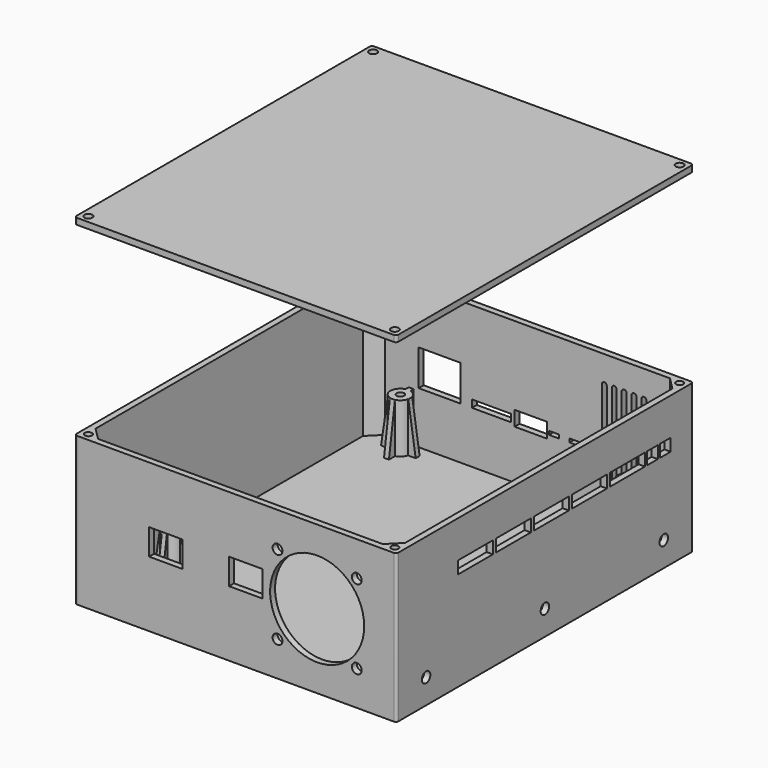
from build123d import *

# Parameters (mm, degrees)
F0_R        = 1.5
F1_DEPTH    = 60
F2_T        = -2.5
F3_DEPTH    = 22.5
F4_W        = 17
F4_H        = 14.5
F4_W_2      = 15.8
F4_H_2      = 3
F4_W_3      = 13
F4_H_3      = 6
F4_W_4      = 4
F4_H_4      = 1.45
F5_DEPTH    = 2.5
F6_R        = 19
F6_R_2      = 2
F6_W        = 13.5
F6_H        = 10.5
F7_DEPTH    = 2.5
F8_R        = 2.15
F8_W        = 17.7
F8_H        = 5
F8_W_2      = 5.5
F9_DEPTH    = 2.5
F12_DEPTH   = 2.5
F13_SIZE2   = 19.99999
F13_SIZE    = 2.99999
F14_SIZE2   = 2.99999
F14_SIZE    = 19.99999
F14_2_SIZE2 = 2.99999
F14_2_SIZE  = 19.99999
F14_3_SIZE2 = 2.99999
F14_3_SIZE  = 19.99999
F14_4_SIZE2 = 2.99999
F14_4_SIZE  = 19.99999
F14_5_SIZE2 = 2.99999
F14_5_SIZE  = 19.99999
F14_6_SIZE2 = 2.99999
F14_6_SIZE  = 19.99999
F14_7_SIZE2 = 2.99999
F14_7_SIZE  = 19.99999
F15_SIZE2   = 19.99999
F15_SIZE    = 2.99999
F15_2_SIZE2 = 19.99999
F15_2_SIZE  = 2.99999
F16_DEPTH   = 60
F17_R       = 1.45
F18_DEPTH   = 15
F19_W       = 130
F19_H       = 150
F20_DEPTH   = 2.5
F22_R       = 1.6
F23_DEPTH   = 2.5
F24_R       = 1
F24_2_R     = 1


# Not quite as in the source:
# - a fillet or chamfer is up to 0.001 mm smaller than in the source, because OpenCascade refuses the exact size


with BuildPart() as f1:
    # F0 (on Top) → F1 (new body)
    with BuildSketch(Plane.XY):
        Polygon((-55, -75), (55, -75), (65, -65), (65, 65), (55, 75), (-55, 75), (-65, 65), (-65, -65), align=None)
        with BuildLine():
            ThreePointArc((-46, -44.1270166538), (-44.1715728753, -45.1715728753), (-43.1270166538, -47))
            Line((-43.1270166538, -47), (-40, -47))
            Line((-40, -47), (-40, -49))
            Line((-40, -49), (-43.1270166538, -49))
            ThreePointArc((-43.1270166538, -49), (-44.1715728753, -50.8284271247), (-46, -51.8729833462))
            Line((-46, -51.8729833462), (-46, -55))
            Line((-46, -55), (-48, -55))
            Line((-48, -55), (-48, -51.8729833462))
            ThreePointArc((-48, -51.8729833462), (-49.8284271247, -50.8284271247), (-50.8729833462, -49))
            Line((-50.8729833462, -49), (-54, -49))
            Line((-54, -49), (-54, -47))
            Line((-54, -47), (-50.8729833462, -47))
            ThreePointArc((-50.8729833462, -47), (-49.8284271247, -45.1715728753), (-48, -44.1270166538))
            Line((-48, -44.1270166538), (-48, -41))
            Line((-48, -41), (-46, -41))
            Line((-46, -41), (-46, -44.1270166538))
        make_face(mode=Mode.SUBTRACT)
        with BuildLine():
            ThreePointArc((46, -44.1270166538), (47.8284271247, -45.1715728753), (48.8729833462, -47))
            Line((48.8729833462, -47), (52, -47))
            Line((52, -47), (52, -49))
            Line((52, -49), (48.8729833462, -49))
            ThreePointArc((48.8729833462, -49), (47.8284271247, -50.8284271247), (46, -51.8729833462))
            Line((46, -51.8729833462), (46, -55))
            Line((46, -55), (44, -55))
            Line((44, -55), (44, -51.8729833462))
            ThreePointArc((44, -51.8729833462), (42.1715728753, -50.8284271247), (41.1270166538, -49))
            Line((41.1270166538, -49), (38, -49))
            Line((38, -49), (38, -47))
            Line((38, -47), (41.1270166538, -47))
            ThreePointArc((41.1270166538, -47), (42.1715728753, -45.1715728753), (44, -44.1270166538))
            Line((44, -44.1270166538), (44, -41))
            Line((44, -41), (46, -41))
            Line((46, -41), (46, -44.1270166538))
        make_face(mode=Mode.SUBTRACT)
        with BuildLine():
            ThreePointArc((-46, 70.8729833462), (-44.1715728753, 69.8284271247), (-43.1270166538, 68))
            Line((-43.1270166538, 68), (-40, 68))
            Line((-40, 68), (-40, 66))
            Line((-40, 66), (-43.1270166538, 66))
            ThreePointArc((-43.1270166538, 66), (-44.1715728753, 64.1715728753), (-46, 63.1270166538))
            Line((-46, 63.1270166538), (-46, 60))
            Line((-46, 60), (-48, 60))
            Line((-48, 60), (-48, 63.1270166538))
            ThreePointArc((-48, 63.1270166538), (-49.8284271247, 64.1715728753), (-50.8729833462, 66))
            Line((-50.8729833462, 66), (-54, 66))
            Line((-54, 66), (-54, 68))
            Line((-54, 68), (-50.8729833462, 68))
            ThreePointArc((-50.8729833462, 68), (-49.8284271247, 69.8284271247), (-48, 70.8729833462))
            Line((-48, 70.8729833462), (-48, 74))
            Line((-48, 74), (-46, 74))
            Line((-46, 74), (-46, 70.8729833462))
        make_face(mode=Mode.SUBTRACT)
        with BuildLine():
            ThreePointArc((46, 70.8729833462), (47.8284271247, 69.8284271247), (48.8729833462, 68))
            Line((48.8729833462, 68), (52, 68))
            Line((52, 68), (52, 66))
            Line((52, 66), (48.8729833462, 66))
            ThreePointArc((48.8729833462, 66), (47.8284271247, 64.1715728753), (46, 63.1270166538))
            Line((46, 63.1270166538), (46, 60))
            Line((46, 60), (44, 60))
            Line((44, 60), (44, 63.1270166538))
            ThreePointArc((44, 63.1270166538), (42.1715728753, 64.1715728753), (41.1270166538, 66))
            Line((41.1270166538, 66), (38, 66))
            Line((38, 66), (38, 68))
            Line((38, 68), (41.1270166538, 68))
            ThreePointArc((41.1270166538, 68), (42.1715728753, 69.8284271247), (44, 70.8729833462))
            Line((44, 70.8729833462), (44, 74))
            Line((44, 74), (46, 74))
            Line((46, 74), (46, 70.8729833462))
        make_face(mode=Mode.SUBTRACT)
        with BuildLine():
            ThreePointArc((48.8729833462, 66), (48.9681187851, 66.4959828301), (49, 67))
            ThreePointArc((49, 67), (48.9681187851, 67.5040171699), (48.8729833462, 68))
            ThreePointArc((48.8729833462, 68), (47.8284271247, 69.8284271247), (46, 70.8729833462))
            ThreePointArc((46, 70.8729833462), (45, 71), (44, 70.8729833462))
            ThreePointArc((44, 70.8729833462), (42.1715728753, 69.8284271247), (41.1270166538, 68))
            ThreePointArc((41.1270166538, 68), (41, 67), (41.1270166538, 66))
            ThreePointArc((41.1270166538, 66), (42.1715728753, 64.1715728753), (44, 63.1270166538))
            ThreePointArc((44, 63.1270166538), (45, 63), (46, 63.1270166538))
            ThreePointArc((46, 63.1270166538), (47.8284271247, 64.1715728753), (48.8729833462, 66))
        make_face()
        with Locations((45, 67)):
            Circle(F0_R, mode=Mode.SUBTRACT)
        with BuildLine():
            ThreePointArc((-43.1270166538, -49), (-43.0318812149, -48.5040171699), (-43, -48))
            ThreePointArc((-43, -48), (-43.0318812149, -47.4959828301), (-43.1270166538, -47))
            ThreePointArc((-43.1270166538, -47), (-44.1715728753, -45.1715728753), (-46, -44.1270166538))
            ThreePointArc((-46, -44.1270166538), (-47, -44), (-48, -44.1270166538))
            ThreePointArc((-48, -44.1270166538), (-49.8284271247, -45.1715728753), (-50.8729833462, -47))
            ThreePointArc((-50.8729833462, -47), (-51, -48), (-50.8729833462, -49))
            ThreePointArc((-50.8729833462, -49), (-49.8284271247, -50.8284271247), (-48, -51.8729833462))
            ThreePointArc((-48, -51.8729833462), (-47, -52), (-46, -51.8729833462))
            ThreePointArc((-46, -51.8729833462), (-44.1715728753, -50.8284271247), (-43.1270166538, -49))
        make_face()
        with Locations((-47, -48)):
            Circle(F0_R, mode=Mode.SUBTRACT)
        with BuildLine():
            ThreePointArc((-43.1270166538, 66), (-43.0318812149, 66.4959828301), (-43, 67))
            ThreePointArc((-43, 67), (-43.0318812149, 67.5040171699), (-43.1270166538, 68))
            ThreePointArc((-43.1270166538, 68), (-44.1715728753, 69.8284271247), (-46, 70.8729833462))
            ThreePointArc((-46, 70.8729833462), (-47, 71), (-48, 70.8729833462))
            ThreePointArc((-48, 70.8729833462), (-49.8284271247, 69.8284271247), (-50.8729833462, 68))
            ThreePointArc((-50.8729833462, 68), (-51, 67), (-50.8729833462, 66))
            ThreePointArc((-50.8729833462, 66), (-49.8284271247, 64.1715728753), (-48, 63.1270166538))
            ThreePointArc((-48, 63.1270166538), (-47, 63), (-46, 63.1270166538))
            ThreePointArc((-46, 63.1270166538), (-44.1715728753, 64.1715728753), (-43.1270166538, 66))
        make_face()
        with Locations((-47, 67)):
            Circle(F0_R, mode=Mode.SUBTRACT)
        with BuildLine():
            ThreePointArc((48.8729833462, -49), (48.9681187851, -48.5040171699), (49, -48))
            ThreePointArc((49, -48), (48.9681187851, -47.4959828301), (48.8729833462, -47))
            ThreePointArc((48.8729833462, -47), (47.8284271247, -45.1715728753), (46, -44.1270166538))
            ThreePointArc((46, -44.1270166538), (45, -44), (44, -44.1270166538))
            ThreePointArc((44, -44.1270166538), (42.1715728753, -45.1715728753), (41.1270166538, -47))
            ThreePointArc((41.1270166538, -47), (41, -48), (41.1270166538, -49))
            ThreePointArc((41.1270166538, -49), (42.1715728753, -50.8284271247), (44, -51.8729833462))
            ThreePointArc((44, -51.8729833462), (45, -52), (46, -51.8729833462))
            ThreePointArc((46, -51.8729833462), (47.8284271247, -50.8284271247), (48.8729833462, -49))
        make_face()
        with Locations((45, -48)):
            Circle(F0_R, mode=Mode.SUBTRACT)
        Polygon((55, -75), (65, -75), (65, -65), align=None)
        Polygon((-65, -75), (-55, -75), (-65, -65), align=None)
        Polygon((55, 75), (65, 65), (65, 75), align=None)
        Polygon((-65, 75), (-65, 65), (-55, 75), align=None)
        with Locations((45, 67)):
            Circle(F0_R)
        with Locations((-47, 67)):
            Circle(F0_R)
        with Locations((-47, -48)):
            Circle(F0_R)
        with Locations((45, -48)):
            Circle(F0_R)
        with BuildLine():
            Line((-46, 60), (-46, 63.1270166538))
            ThreePointArc((-46, 63.1270166538), (-47, 63), (-48, 63.1270166538))
            Line((-48, 63.1270166538), (-48, 60))
            Line((-48, 60), (-46, 60))
        make_face()
        with BuildLine():
            ThreePointArc((-50.8729833462, -49), (-51, -48), (-50.8729833462, -47))
            Line((-50.8729833462, -47), (-54, -47))
            Line((-54, -47), (-54, -49))
            Line((-54, -49), (-50.8729833462, -49))
        make_face()
        with BuildLine():
            Line((-46, -55), (-46, -51.8729833462))
            ThreePointArc((-46, -51.8729833462), (-47, -52), (-48, -51.8729833462))
            Line((-48, -51.8729833462), (-48, -55))
            Line((-48, -55), (-46, -55))
        make_face()
        with BuildLine():
            ThreePointArc((-50.8729833462, 66), (-51, 67), (-50.8729833462, 68))
            Line((-50.8729833462, 68), (-54, 68))
            Line((-54, 68), (-54, 66))
            Line((-54, 66), (-50.8729833462, 66))
        make_face()
        with BuildLine():
            Line((46, -55), (46, -51.8729833462))
            ThreePointArc((46, -51.8729833462), (45, -52), (44, -51.8729833462))
            Line((44, -51.8729833462), (44, -55))
            Line((44, -55), (46, -55))
        make_face()
        with BuildLine():
            ThreePointArc((48.8729833462, 68), (48.9681187851, 67.5040171699), (49, 67))
            ThreePointArc((49, 67), (48.9681187851, 66.4959828301), (48.8729833462, 66))
            Line((48.8729833462, 66), (52, 66))
            Line((52, 66), (52, 68))
            Line((52, 68), (48.8729833462, 68))
        make_face()
        with BuildLine():
            Line((46, 60), (46, 63.1270166538))
            ThreePointArc((46, 63.1270166538), (45, 63), (44, 63.1270166538))
            Line((44, 63.1270166538), (44, 60))
            Line((44, 60), (46, 60))
        make_face()
        with BuildLine():
            ThreePointArc((-43.1270166538, -47), (-43.0318812149, -47.4959828301), (-43, -48))
            ThreePointArc((-43, -48), (-43.0318812149, -48.5040171699), (-43.1270166538, -49))
            Line((-43.1270166538, -49), (-40, -49))
            Line((-40, -49), (-40, -47))
            Line((-40, -47), (-43.1270166538, -47))
        make_face()
        with BuildLine():
            ThreePointArc((44, -44.1270166538), (45, -44), (46, -44.1270166538))
            Line((46, -44.1270166538), (46, -41))
            Line((46, -41), (44, -41))
            Line((44, -41), (44, -44.1270166538))
        make_face()
        with BuildLine():
            ThreePointArc((41.1270166538, -49), (41, -48), (41.1270166538, -47))
            Line((41.1270166538, -47), (38, -47))
            Line((38, -47), (38, -49))
            Line((38, -49), (41.1270166538, -49))
        make_face()
        with BuildLine():
            ThreePointArc((-48, -44.1270166538), (-47, -44), (-46, -44.1270166538))
            Line((-46, -44.1270166538), (-46, -41))
            Line((-46, -41), (-48, -41))
            Line((-48, -41), (-48, -44.1270166538))
        make_face()
        with BuildLine():
            ThreePointArc((-43.1270166538, 68), (-43.0318812149, 67.5040171699), (-43, 67))
            ThreePointArc((-43, 67), (-43.0318812149, 66.4959828301), (-43.1270166538, 66))
            Line((-43.1270166538, 66), (-40, 66))
            Line((-40, 66), (-40, 68))
            Line((-40, 68), (-43.1270166538, 68))
        make_face()
        with BuildLine():
            ThreePointArc((44, 70.8729833462), (45, 71), (46, 70.8729833462))
            Line((46, 70.8729833462), (46, 74))
            Line((46, 74), (44, 74))
            Line((44, 74), (44, 70.8729833462))
        make_face()
        with BuildLine():
            ThreePointArc((48.8729833462, -47), (48.9681187851, -47.4959828301), (49, -48))
            ThreePointArc((49, -48), (48.9681187851, -48.5040171699), (48.8729833462, -49))
            Line((48.8729833462, -49), (52, -49))
            Line((52, -49), (52, -47))
            Line((52, -47), (48.8729833462, -47))
        make_face()
        with BuildLine():
            ThreePointArc((41.1270166538, 66), (41, 67), (41.1270166538, 68))
            Line((41.1270166538, 68), (38, 68))
            Line((38, 68), (38, 66))
            Line((38, 66), (41.1270166538, 66))
        make_face()
        with BuildLine():
            ThreePointArc((-48, 70.8729833462), (-47, 71), (-46, 70.8729833462))
            Line((-46, 70.8729833462), (-46, 74))
            Line((-46, 74), (-48, 74))
            Line((-48, 74), (-48, 70.8729833462))
        make_face()
    extrude(amount=F1_DEPTH)

    # F2
    f2_openings = [f1.faces().sort_by_distance(p)[0] for p in [
        (0, 0, 60),
    ]]
    offset(amount=F2_T, openings=f2_openings)

    # F0 (on Top) → F3 (join)
    with BuildSketch(Plane.XY):
        with BuildLine():
            ThreePointArc((-43.1270166538, 66), (-43.0318812149, 66.4959828301), (-43, 67))
            ThreePointArc((-43, 67), (-43.0318812149, 67.5040171699), (-43.1270166538, 68))
            ThreePointArc((-43.1270166538, 68), (-44.1715728753, 69.8284271247), (-46, 70.8729833462))
            ThreePointArc((-46, 70.8729833462), (-47, 71), (-48, 70.8729833462))
            ThreePointArc((-48, 70.8729833462), (-49.8284271247, 69.8284271247), (-50.8729833462, 68))
            ThreePointArc((-50.8729833462, 68), (-51, 67), (-50.8729833462, 66))
            ThreePointArc((-50.8729833462, 66), (-49.8284271247, 64.1715728753), (-48, 63.1270166538))
            ThreePointArc((-48, 63.1270166538), (-47, 63), (-46, 63.1270166538))
            ThreePointArc((-46, 63.1270166538), (-44.1715728753, 64.1715728753), (-43.1270166538, 66))
        make_face()
        with Locations((-47, 67)):
            Circle(F0_R, mode=Mode.SUBTRACT)
        with BuildLine():
            ThreePointArc((-43.1270166538, -49), (-43.0318812149, -48.5040171699), (-43, -48))
            ThreePointArc((-43, -48), (-43.0318812149, -47.4959828301), (-43.1270166538, -47))
            ThreePointArc((-43.1270166538, -47), (-44.1715728753, -45.1715728753), (-46, -44.1270166538))
            ThreePointArc((-46, -44.1270166538), (-47, -44), (-48, -44.1270166538))
            ThreePointArc((-48, -44.1270166538), (-49.8284271247, -45.1715728753), (-50.8729833462, -47))
            ThreePointArc((-50.8729833462, -47), (-51, -48), (-50.8729833462, -49))
            ThreePointArc((-50.8729833462, -49), (-49.8284271247, -50.8284271247), (-48, -51.8729833462))
            ThreePointArc((-48, -51.8729833462), (-47, -52), (-46, -51.8729833462))
            ThreePointArc((-46, -51.8729833462), (-44.1715728753, -50.8284271247), (-43.1270166538, -49))
        make_face()
        with Locations((-47, -48)):
            Circle(F0_R, mode=Mode.SUBTRACT)
        with BuildLine():
            ThreePointArc((48.8729833462, -49), (48.9681187851, -48.5040171699), (49, -48))
            ThreePointArc((49, -48), (48.9681187851, -47.4959828301), (48.8729833462, -47))
            ThreePointArc((48.8729833462, -47), (47.8284271247, -45.1715728753), (46, -44.1270166538))
            ThreePointArc((46, -44.1270166538), (45, -44), (44, -44.1270166538))
            ThreePointArc((44, -44.1270166538), (42.1715728753, -45.1715728753), (41.1270166538, -47))
            ThreePointArc((41.1270166538, -47), (41, -48), (41.1270166538, -49))
            ThreePointArc((41.1270166538, -49), (42.1715728753, -50.8284271247), (44, -51.8729833462))
            ThreePointArc((44, -51.8729833462), (45, -52), (46, -51.8729833462))
            ThreePointArc((46, -51.8729833462), (47.8284271247, -50.8284271247), (48.8729833462, -49))
        make_face()
        with Locations((45, -48)):
            Circle(F0_R, mode=Mode.SUBTRACT)
        with BuildLine():
            ThreePointArc((48.8729833462, 66), (48.9681187851, 66.4959828301), (49, 67))
            ThreePointArc((49, 67), (48.9681187851, 67.5040171699), (48.8729833462, 68))
            ThreePointArc((48.8729833462, 68), (47.8284271247, 69.8284271247), (46, 70.8729833462))
            ThreePointArc((46, 70.8729833462), (45, 71), (44, 70.8729833462))
            ThreePointArc((44, 70.8729833462), (42.1715728753, 69.8284271247), (41.1270166538, 68))
            ThreePointArc((41.1270166538, 68), (41, 67), (41.1270166538, 66))
            ThreePointArc((41.1270166538, 66), (42.1715728753, 64.1715728753), (44, 63.1270166538))
            ThreePointArc((44, 63.1270166538), (45, 63), (46, 63.1270166538))
            ThreePointArc((46, 63.1270166538), (47.8284271247, 64.1715728753), (48.8729833462, 66))
        make_face()
        with Locations((45, 67)):
            Circle(F0_R, mode=Mode.SUBTRACT)
        with BuildLine():
            ThreePointArc((48.8729833462, 68), (48.9681187851, 67.5040171699), (49, 67))
            ThreePointArc((49, 67), (48.9681187851, 66.4959828301), (48.8729833462, 66))
            Line((48.8729833462, 66), (52, 66))
            Line((52, 66), (52, 68))
            Line((52, 68), (48.8729833462, 68))
        make_face()
        with BuildLine():
            Line((46, 60), (46, 63.1270166538))
            ThreePointArc((46, 63.1270166538), (45, 63), (44, 63.1270166538))
            Line((44, 63.1270166538), (44, 60))
            Line((44, 60), (46, 60))
        make_face()
        with BuildLine():
            ThreePointArc((41.1270166538, 66), (41, 67), (41.1270166538, 68))
            Line((41.1270166538, 68), (38, 68))
            Line((38, 68), (38, 66))
            Line((38, 66), (41.1270166538, 66))
        make_face()
        with BuildLine():
            ThreePointArc((44, 70.8729833462), (45, 71), (46, 70.8729833462))
            Line((46, 70.8729833462), (46, 74))
            Line((46, 74), (44, 74))
            Line((44, 74), (44, 70.8729833462))
        make_face()
        with BuildLine():
            ThreePointArc((-48, 70.8729833462), (-47, 71), (-46, 70.8729833462))
            Line((-46, 70.8729833462), (-46, 74))
            Line((-46, 74), (-48, 74))
            Line((-48, 74), (-48, 70.8729833462))
        make_face()
        with BuildLine():
            ThreePointArc((-50.8729833462, 66), (-51, 67), (-50.8729833462, 68))
            Line((-50.8729833462, 68), (-54, 68))
            Line((-54, 68), (-54, 66))
            Line((-54, 66), (-50.8729833462, 66))
        make_face()
        with BuildLine():
            Line((-46, 60), (-46, 63.1270166538))
            ThreePointArc((-46, 63.1270166538), (-47, 63), (-48, 63.1270166538))
            Line((-48, 63.1270166538), (-48, 60))
            Line((-48, 60), (-46, 60))
        make_face()
        with BuildLine():
            ThreePointArc((-43.1270166538, 68), (-43.0318812149, 67.5040171699), (-43, 67))
            ThreePointArc((-43, 67), (-43.0318812149, 66.4959828301), (-43.1270166538, 66))
            Line((-43.1270166538, 66), (-40, 66))
            Line((-40, 66), (-40, 68))
            Line((-40, 68), (-43.1270166538, 68))
        make_face()
        with BuildLine():
            ThreePointArc((-43.1270166538, -47), (-43.0318812149, -47.4959828301), (-43, -48))
            ThreePointArc((-43, -48), (-43.0318812149, -48.5040171699), (-43.1270166538, -49))
            Line((-43.1270166538, -49), (-40, -49))
            Line((-40, -49), (-40, -47))
            Line((-40, -47), (-43.1270166538, -47))
        make_face()
        with BuildLine():
            ThreePointArc((-48, -44.1270166538), (-47, -44), (-46, -44.1270166538))
            Line((-46, -44.1270166538), (-46, -41))
            Line((-46, -41), (-48, -41))
            Line((-48, -41), (-48, -44.1270166538))
        make_face()
        with BuildLine():
            ThreePointArc((-50.8729833462, -49), (-51, -48), (-50.8729833462, -47))
            Line((-50.8729833462, -47), (-54, -47))
            Line((-54, -47), (-54, -49))
            Line((-54, -49), (-50.8729833462, -49))
        make_face()
        with BuildLine():
            Line((-46, -55), (-46, -51.8729833462))
            ThreePointArc((-46, -51.8729833462), (-47, -52), (-48, -51.8729833462))
            Line((-48, -51.8729833462), (-48, -55))
            Line((-48, -55), (-46, -55))
        make_face()
        with BuildLine():
            ThreePointArc((41.1270166538, -49), (41, -48), (41.1270166538, -47))
            Line((41.1270166538, -47), (38, -47))
            Line((38, -47), (38, -49))
            Line((38, -49), (41.1270166538, -49))
        make_face()
        with BuildLine():
            ThreePointArc((44, -44.1270166538), (45, -44), (46, -44.1270166538))
            Line((46, -44.1270166538), (46, -41))
            Line((46, -41), (44, -41))
            Line((44, -41), (44, -44.1270166538))
        make_face()
        with BuildLine():
            ThreePointArc((48.8729833462, -47), (48.9681187851, -47.4959828301), (49, -48))
            ThreePointArc((49, -48), (48.9681187851, -48.5040171699), (48.8729833462, -49))
            Line((48.8729833462, -49), (52, -49))
            Line((52, -49), (52, -47))
            Line((52, -47), (48.8729833462, -47))
        make_face()
        with BuildLine():
            Line((46, -55), (46, -51.8729833462))
            ThreePointArc((46, -51.8729833462), (45, -52), (44, -51.8729833462))
            Line((44, -51.8729833462), (44, -55))
            Line((44, -55), (46, -55))
        make_face()
    extrude(amount=F3_DEPTH)

    # F4 (on face) → F5 (cut, through all)
    with BuildSketch(Plane(origin=(0, 75, 0), x_dir=(-1, 0, 0), z_dir=(0, 1, 0))):
        with Locations((35.5, 30.75)):
            Rectangle(F4_W, F4_H)
        with Locations((14.6, 25)):
            Rectangle(F4_W_2, F4_H_2)
        with Locations((-1.25, 25.4)):
            Rectangle(F4_W_3, F4_H_3)
        with Locations((-10.65, 24.725)):
            Rectangle(F4_W_4, F4_H_4)
        with Locations((-18.95, 24.725)):
            Rectangle(F4_W_4, F4_H_4)
    extrude(amount=-F5_DEPTH, mode=Mode.SUBTRACT)

    # F6 (on face) → F7 (cut, through all)
    with BuildSketch(Plane.XZ.offset(75)):
        with Locations((33, 30)):
            Circle(F6_R)
        with Locations((17, 46)):
            Circle(F6_R_2)
        with Locations((49, 46)):
            Circle(F6_R_2)
        with Locations((49, 14)):
            Circle(F6_R_2)
        with Locations((17, 14)):
            Circle(F6_R_2)
        with Locations((4.125, 31.75)):
            Rectangle(F6_W, F6_H)
        with Locations((-28.125, 31.75)):
            Rectangle(F6_W, F6_H)
    extrude(amount=-F7_DEPTH, mode=Mode.SUBTRACT)

    # F8 (on face) → F9 (cut, through all)
    with BuildSketch(Plane.YZ.offset(65)):
        with Locations((-60, 10)):
            Circle(F8_R)
        with Locations((60, 10)):
            Circle(F8_R)
        with Locations((0, 10)):
            Circle(F8_R)
        with Locations((-35.15, 42.5)):
            Rectangle(F8_W, F8_H)
        with Locations((60.75, 42.5)):
            Rectangle(F8_W_2, F8_H)
        with Locations((54.25, 42.5)):
            Rectangle(F8_W_2, F8_H)
        with Locations((41.65, 42.5)):
            Rectangle(F8_W, F8_H)
        with Locations((22.45, 42.5)):
            Rectangle(F8_W, F8_H)
        with Locations((3.25, 42.5)):
            Rectangle(F8_W, F8_H)
        with Locations((-15.95, 42.5)):
            Rectangle(F8_W, F8_H)
    extrude(amount=-F9_DEPTH, mode=Mode.SUBTRACT)

    # F11 (on face) → F12 (cut, through all)
    with BuildSketch(Plane(origin=(0, 75, 0), x_dir=(-1, 0, 0), z_dir=(0, 1, 0))):
        with BuildLine():
            ThreePointArc((-51, 50), (-51.7071067812, 49.7071067812), (-52, 49))
            Line((-52, 49), (-52, 11))
            ThreePointArc((-52, 11), (-51.7071067812, 10.2928932188), (-51, 10))
            ThreePointArc((-51, 10), (-50.2928932188, 10.2928932188), (-50, 11))
            Line((-50, 11), (-50, 49))
            ThreePointArc((-50, 49), (-50.2928932188, 49.7071067812), (-51, 50))
        make_face()
        with BuildLine():
            ThreePointArc((-47, 50), (-47.7071067812, 49.7071067812), (-48, 49))
            Line((-48, 49), (-48, 11))
            ThreePointArc((-48, 11), (-47.7071067812, 10.2928932188), (-47, 10))
            ThreePointArc((-47, 10), (-46.2928932188, 10.2928932188), (-46, 11))
            Line((-46, 11), (-46, 49))
            ThreePointArc((-46, 49), (-46.2928932188, 49.7071067812), (-47, 50))
        make_face()
        with BuildLine():
            ThreePointArc((-43, 50), (-43.7071067812, 49.7071067812), (-44, 49))
            Line((-44, 49), (-44, 11))
            ThreePointArc((-44, 11), (-43.7071067812, 10.2928932188), (-43, 10))
            ThreePointArc((-43, 10), (-42.2928932188, 10.2928932188), (-42, 11))
            Line((-42, 11), (-42, 49))
            ThreePointArc((-42, 49), (-42.2928932188, 49.7071067812), (-43, 50))
        make_face()
        with BuildLine():
            ThreePointArc((-39, 50), (-39.7071067812, 49.7071067812), (-40, 49))
            Line((-40, 49), (-40, 11))
            ThreePointArc((-40, 11), (-39.7071067812, 10.2928932188), (-39, 10))
            ThreePointArc((-39, 10), (-38.2928932188, 10.2928932188), (-38, 11))
            Line((-38, 11), (-38, 49))
            ThreePointArc((-38, 49), (-38.2928932188, 49.7071067812), (-39, 50))
        make_face()
        with BuildLine():
            ThreePointArc((-35, 50), (-35.7071067812, 49.7071067812), (-36, 49))
            Line((-36, 49), (-36, 11))
            ThreePointArc((-36, 11), (-35.7071067812, 10.2928932188), (-35, 10))
            ThreePointArc((-35, 10), (-34.2928932188, 10.2928932188), (-34, 11))
            Line((-34, 11), (-34, 49))
            ThreePointArc((-34, 49), (-34.2928932188, 49.7071067812), (-35, 50))
        make_face()
        with BuildLine():
            ThreePointArc((-31, 50), (-31.7071067812, 49.7071067812), (-32, 49))
            Line((-32, 49), (-32, 11))
            ThreePointArc((-32, 11), (-31.7071067812, 10.2928932188), (-31, 10))
            ThreePointArc((-31, 10), (-30.2928932188, 10.2928932188), (-30, 11))
            Line((-30, 11), (-30, 49))
            ThreePointArc((-30, 49), (-30.2928932188, 49.7071067812), (-31, 50))
        make_face()
    extrude(amount=-F12_DEPTH, mode=Mode.SUBTRACT)

    # F13 (size 3 and 20 in the source; OpenCascade refuses exactly that, so slightly less here)
    f13_edges = [f1.edges().sort_by_distance(p)[0] for p in [
        (-40, -48, 22.5),
        (-47, -41, 22.5),
        (-54, -48, 22.5),
        (-47, -55, 22.5),
    ]]
    f13_side = f1.faces().sort_by_distance((-44.311573, -45.311573, 22.5))[0]
    chamfer(f13_edges, length=F13_SIZE, length2=F13_SIZE2, reference=f13_side)

    # F14 (size 20 and 3 in the source; OpenCascade refuses exactly that, so slightly less here)
    f14_edges = [f1.edges().sort_by_distance(p)[0] for p in [
        (-47, 60, 22.5),
    ]]
    f14_side = f1.faces().sort_by_distance((-47, 60, 12.5))[0]
    chamfer(f14_edges, length=F14_SIZE, length2=F14_SIZE2, reference=f14_side)

    # F14#2 (size 20 and 3 in the source; OpenCascade refuses exactly that, so slightly less here)
    f14_2_edges = [f1.edges().sort_by_distance(p)[0] for p in [
        (-40, 67, 22.5),
    ]]
    f14_2_side = f1.faces().sort_by_distance((-40, 67, 12.5))[0]
    chamfer(f14_2_edges, length=F14_2_SIZE, length2=F14_2_SIZE2, reference=f14_2_side)

    # F14#3 (size 20 and 3 in the source; OpenCascade refuses exactly that, so slightly less here)
    f14_3_edges = [f1.edges().sort_by_distance(p)[0] for p in [
        (-54, 67, 22.5),
    ]]
    f14_3_side = f1.faces().sort_by_distance((-54, 67, 12.5))[0]
    chamfer(f14_3_edges, length=F14_3_SIZE, length2=F14_3_SIZE2, reference=f14_3_side)

    # F14#4 (size 20 and 3 in the source; OpenCascade refuses exactly that, so slightly less here)
    f14_4_edges = [f1.edges().sort_by_distance(p)[0] for p in [
        (45, 60, 22.5),
    ]]
    f14_4_side = f1.faces().sort_by_distance((45, 60, 12.5))[0]
    chamfer(f14_4_edges, length=F14_4_SIZE, length2=F14_4_SIZE2, reference=f14_4_side)

    # F14#5 (size 20 and 3 in the source; OpenCascade refuses exactly that, so slightly less here)
    f14_5_edges = [f1.edges().sort_by_distance(p)[0] for p in [
        (38, 67, 22.5),
    ]]
    f14_5_side = f1.faces().sort_by_distance((38, 67, 12.5))[0]
    chamfer(f14_5_edges, length=F14_5_SIZE, length2=F14_5_SIZE2, reference=f14_5_side)

    # F14#6 (size 20 and 3 in the source; OpenCascade refuses exactly that, so slightly less here)
    f14_6_edges = [f1.edges().sort_by_distance(p)[0] for p in [
        (38, -48, 22.5),
    ]]
    f14_6_side = f1.faces().sort_by_distance((38, -48, 12.5))[0]
    chamfer(f14_6_edges, length=F14_6_SIZE, length2=F14_6_SIZE2, reference=f14_6_side)

    # F14#7 (size 20 and 3 in the source; OpenCascade refuses exactly that, so slightly less here)
    f14_7_edges = [f1.edges().sort_by_distance(p)[0] for p in [
        (45, -55, 22.5),
    ]]
    f14_7_side = f1.faces().sort_by_distance((45, -55, 12.5))[0]
    chamfer(f14_7_edges, length=F14_7_SIZE, length2=F14_7_SIZE2, reference=f14_7_side)

    # F15 (size 3 and 20 in the source; OpenCascade refuses exactly that, so slightly less here)
    f15_edges = [f1.edges().sort_by_distance(p)[0] for p in [
        (52, -48, 22.5),
        (45, -41, 22.5),
    ]]
    f15_side = f1.faces().sort_by_distance((44.155564, -51.936497, 22.5))[0]
    chamfer(f15_edges, length=F15_SIZE, length2=F15_SIZE2, reference=f15_side)

    # F15#2 (size 3 and 20 in the source; OpenCascade refuses exactly that, so slightly less here)
    f15_2_edges = [f1.edges().sort_by_distance(p)[0] for p in [
        (52, 67, 22.5),
    ]]
    f15_2_side = f1.faces().sort_by_distance((41.063503, 66.145345, 22.5))[0]
    chamfer(f15_2_edges, length=F15_2_SIZE, length2=F15_2_SIZE2, reference=f15_2_side)

    # F0 (on Top) → F16 (join, through all)
    with BuildSketch(Plane.XY):
        Polygon((-65, 75), (-65, 65), (-55, 75), align=None)
        Polygon((-65, -75), (-55, -75), (-65, -65), align=None)
        Polygon((55, -75), (65, -75), (65, -65), align=None)
        Polygon((55, 75), (65, 65), (65, 75), align=None)
    extrude(amount=F16_DEPTH)

    # F17 (on face) → F18 (cut)
    with BuildSketch(Plane.XY.offset(60)):
        with Locations((-61.9, -71.9)):
            Circle(F17_R)
        with Locations((-61.9, 71.9)):
            Circle(F17_R)
        with Locations((61.9, -71.9)):
            Circle(F17_R)
        with Locations((61.9, 71.9)):
            Circle(F17_R)
    extrude(amount=-F18_DEPTH, mode=Mode.SUBTRACT)

    # F24
    f24_edges = [f1.edges().sort_by_distance(p)[0] for p in [
        (65, -75, 30),
        (-65, -75, 30),
        (65, 75, 30),
        (-65, 75, 30),
        (-65, 0, 0),
    ]]
    fillet(f24_edges, radius=F24_R)


with BuildPart() as f20:
    # F19 (on face) → F20 (new body)
    with BuildSketch(Plane.XY.offset(60)):
        Rectangle(F19_W, F19_H)
    extrude(amount=F20_DEPTH)


with BuildPart() as f20_1:
    # F21: moved
    add(f20.part.moved(Location((0, 0, 75))))

    # F22 (on face) → F23 (cut, through all)
    with BuildSketch(Plane.XY.offset(137.5)):
        with Locations((-61.9, -71.9)):
            Circle(F22_R)
        with Locations((61.9, -71.9)):
            Circle(F22_R)
        with Locations((61.9, 71.9)):
            Circle(F22_R)
        with Locations((-61.9, 71.9)):
            Circle(F22_R)
    extrude(amount=-F23_DEPTH, mode=Mode.SUBTRACT)

    # F24#2
    f24_2_edges = [f20_1.edges().sort_by_distance(p)[0] for p in [
        (65, -75, 136.25),
        (65, 75, 136.25),
        (-65, 75, 136.25),
        (-65, -75, 136.25),
    ]]
    fillet(f24_2_edges, radius=F24_2_R)


solid = Compound([f1.part, f20_1.part])
